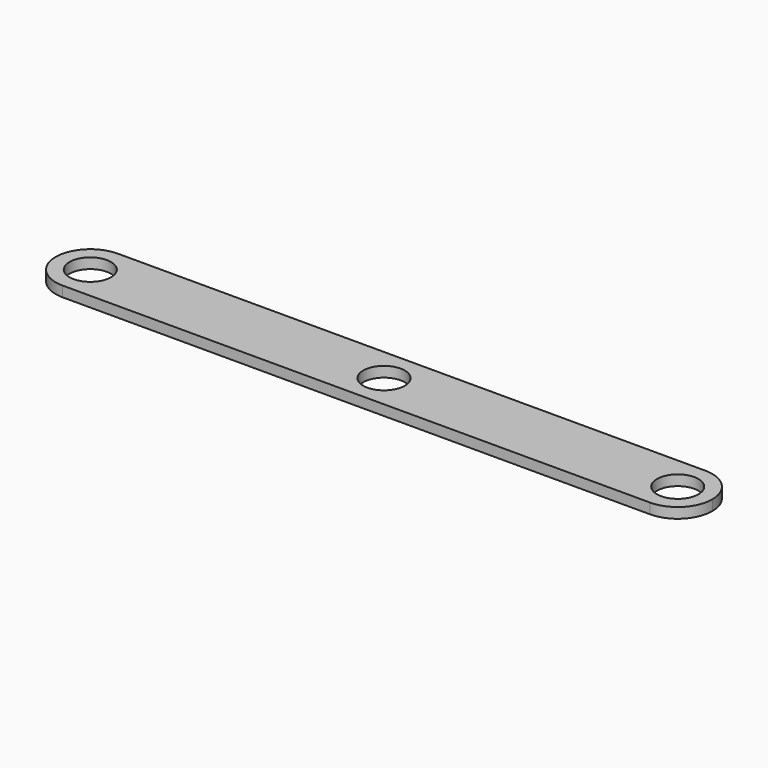
from build123d import *

# Parameters (mm, degrees)
F0_W     = 190
F0_H     = 20
F1_DEPTH = 1.5
F2_R     = 6
F3_DEPTH = 3.001
F4_R     = 6
F5_DEPTH = 3.001
F6_R     = 9.99999


# Not quite as in the source:
# - a fillet or chamfer is up to 0.001 mm smaller than in the source, because OpenCascade refuses the exact size


with BuildPart() as f1:
    # F0 (on Top) → F1 (new body, symmetric)
    with BuildSketch(Plane.XY):
        Rectangle(F0_W, F0_H)
    extrude(amount=F1_DEPTH, both=True)

    # F2 (on face) → F3 (cut, through all)
    with BuildSketch(Plane.XY.offset(1.5)):
        with Locations((-85, 0)):
            Circle(F2_R)
        with Locations((85, 0)):
            Circle(F2_R)
    extrude(amount=-F3_DEPTH, mode=Mode.SUBTRACT)

    # F4 (on face) → F5 (cut, through all)
    with BuildSketch(Plane.XY.offset(1.5)):
        Circle(F4_R)
    extrude(amount=-F5_DEPTH, mode=Mode.SUBTRACT)

    # F6 (radius 10 in the source; OpenCascade refuses exactly that, so slightly less here)
    f6_edges = [f1.edges().sort_by_distance(p)[0] for p in [
        (-95, -10, 0),
        (-95, 10, 0),
        (95, -10, 0),
        (95, 10, 0),
    ]]
    fillet(f6_edges, radius=F6_R)


solid = f1.part
